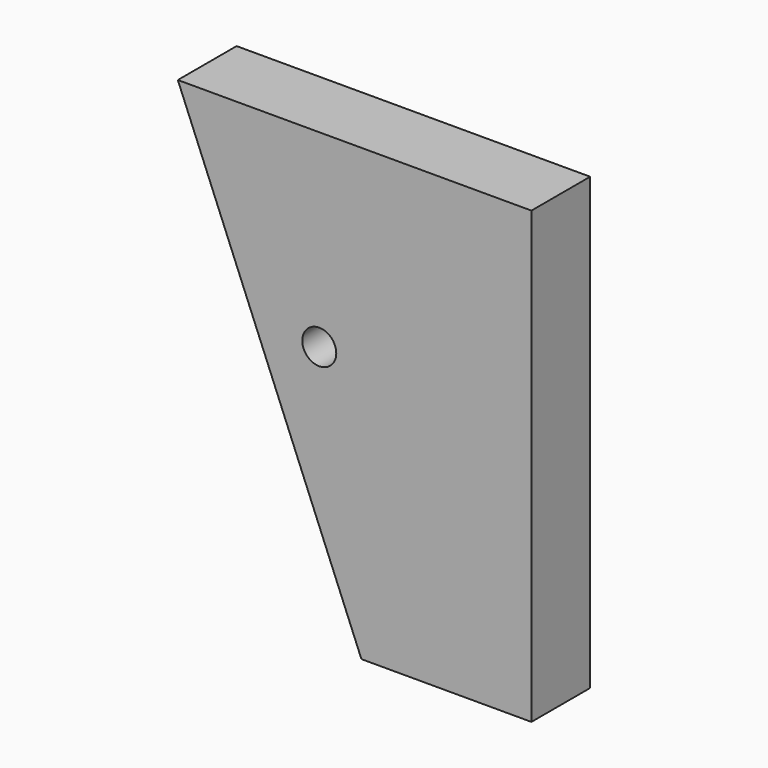
from build123d import *

# Parameters (mm, degrees)
F1_DEPTH = 3.429


with BuildPart() as f1:
    # F0 (on Front) → F1 (new body, symmetric)
    with BuildSketch(Plane.XZ):
        Polygon((20.6095185396, -24.8038658976), (20.6095185396, 17.2331341024), (-12.4104814604, 17.2331341024), (0.7975185396, -15.1509251569), (4.7345185396, -24.8038658976), align=None)
        with BuildLine():
            ThreePointArc((2.3850185396, -0.4198658976), (1.9200505547, -1.5423979128), (0.7975185396, -2.0073658976))
            ThreePointArc((0.7975185396, -2.0073658976), (-0.3250134755, 0.7026661175), (2.3850185396, -0.4198658976))
        make_face(mode=Mode.SUBTRACT)
    extrude(amount=F1_DEPTH, both=True)


solid = f1.part
